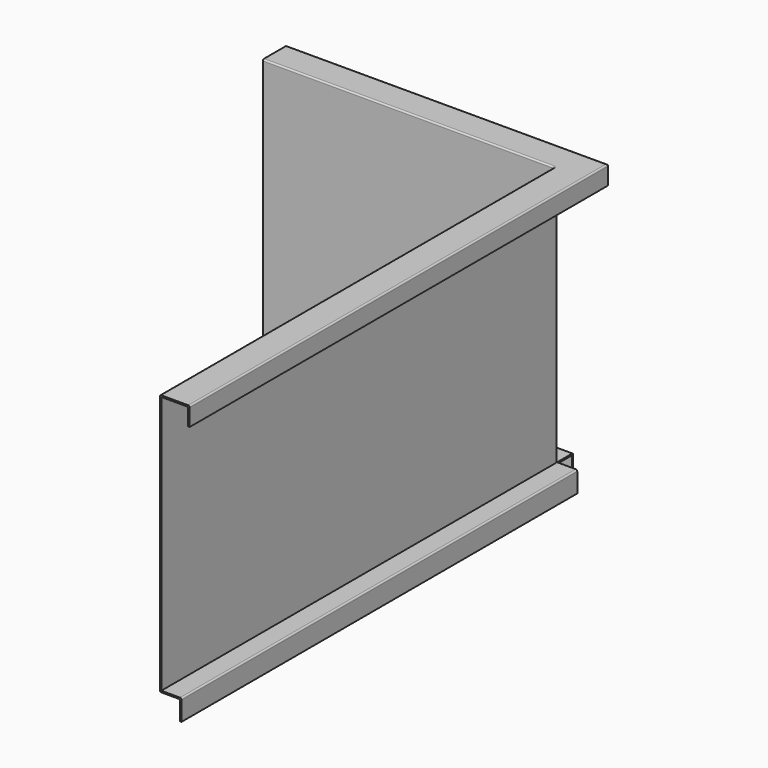
from build123d import *

# Parameters (mm, degrees)
F3_W         = 27
F3_H         = 27
F4_DEPTH     = 30
F5_T1_DEPTH  = 392
F5_T3_DEPTH  = 662
F5_T5_DEPTH  = 350
F5_T10_DEPTH = 703
F5_T15_DEPTH = 433
F5_T17_DEPTH = 672
F5_T19_DEPTH = 402
F5_T21_DEPTH = 440
F5_T23_DEPTH = 710
F5_T25_DEPTH = 346
F5_T27_DEPTH = 660
F5_T29_DEPTH = 390
F5_T32_ANGLE = 90
F5_T33_DEPTH = 663
F5_T35_DEPTH = 393
F5_T38_ANGLE = 90
F5_T40_ANGLE = 90


# Not quite as in the source:
# - a fillet or chamfer that OpenCascade refuses, or shapes differently, is made with other operations: its cross-section is extruded or revolved along the edge and cut away or added


with BuildPart() as f2:
    # F2: sweep along a path in F1
    with BuildLine(Plane.XY) as f2_path:
        Line((0, 0), (0, 660))
        Line((0, 660), (-390, 660))
    # F0 (on Front) → F2 (sweep)
    with BuildSketch(Plane.XZ):
        Polygon((38, -2), (38, -25), (40, -25), (40, 0), (0, 0), (0, -350), (27, -350), (27, -376), (29, -376), (29, -348), (2, -348), (2, -2), align=None)
    sweep(path=f2_path.line, transition=Transition.RIGHT)

    # F3 (on face) → F4 (cut)
    with BuildSketch(Plane.XY.offset(-348)):
        with Locations((15.5, 675.5)):
            Rectangle(F3_W, F3_H)
    extrude(amount=-F4_DEPTH, mode=Mode.SUBTRACT)

    # F5: fillet of radius 2 on 16 edges, made by hand

    # F5_s2 → F5_t1 (join)
    with BuildSketch(Plane.YZ.offset(-390)):
        with BuildLine():
            ThreePointArc((685, -350), (686.4142135624, -350.5857864376), (687, -352))
            Line((687, -352), (687, -350))
            Line((687, -350), (685, -350))
        make_face()
    extrude(amount=F5_T1_DEPTH)

    # F5_s4 → F5_t3 (join)
    with BuildSketch(Plane.XZ.offset(-662)):
        with BuildLine():
            ThreePointArc((25, -350), (26.4142135624, -350.5857864376), (27, -352))
            Line((27, -352), (27, -350))
            Line((27, -350), (25, -350))
        make_face()
    extrude(amount=F5_T3_DEPTH)

    # F5_s6 → F5_t5 (join)
    with BuildSketch(Plane.XY.offset(-350)):
        with BuildLine():
            ThreePointArc((0, 658), (-0.5857864376, 659.4142135624), (-2, 660))
            Line((-2, 660), (0, 660))
            Line((0, 660), (0, 658))
        make_face()
    extrude(amount=F5_T5_DEPTH)


with BuildPart() as f5_tool8:
    # F5_s9 → F5_t10 (new body)
    with BuildSketch(Plane.XZ):
        with BuildLine():
            ThreePointArc((38, -4), (37.4142135624, -2.5857864376), (36, -2))
            Line((36, -2), (38, -2))
            Line((38, -2), (38, -4))
        make_face()
    extrude(amount=-F5_T10_DEPTH)

    split(bisect_by=Plane.XZ.offset(-700), keep=Keep.TOP)


with BuildPart() as f2_1:
    add(f2.part)

    # F5_t7: union F5_tool8
    add(f5_tool8.part)


with BuildPart() as f5_tool13:
    # F5_s14 → F5_t15 (new body)
    with BuildSketch(Plane.YZ.offset(43)):
        with BuildLine():
            ThreePointArc((696, -2), (697.4142135624, -2.5857864376), (698, -4))
            Line((698, -4), (698, -2))
            Line((698, -2), (696, -2))
        make_face()
    extrude(amount=-F5_T15_DEPTH)

    split(bisect_by=Plane.YZ.offset(40), keep=Keep.BOTTOM)


with BuildPart() as f2_2:
    add(f2_1.part)

    # F5_t12: union F5_tool13
    add(f5_tool13.part)

    # F5_s18 → F5_t17 (cut)
    with BuildSketch(Plane.XZ.offset(-667)):
        with BuildLine():
            ThreePointArc((29, -350), (28.4142135624, -348.5857864376), (27, -348))
            Line((27, -348), (29, -348))
            Line((29, -348), (29, -350))
        make_face()
    extrude(amount=F5_T17_DEPTH, mode=Mode.SUBTRACT)

    # F5_s20 → F5_t19 (cut)
    with BuildSketch(Plane.YZ.offset(-395)):
        with BuildLine():
            ThreePointArc((689, -350), (688.4142135624, -348.5857864376), (687, -348))
            Line((687, -348), (689, -348))
            Line((689, -348), (689, -350))
        make_face()
    extrude(amount=F5_T19_DEPTH, mode=Mode.SUBTRACT)

    # F5_s22 → F5_t21 (cut)
    with BuildSketch(Plane.YZ.offset(-395)):
        with BuildLine():
            ThreePointArc((700, -2), (699.4142135624, -0.5857864376), (698, 0))
            Line((698, 0), (700, 0))
            Line((700, 0), (700, -2))
        make_face()
    extrude(amount=F5_T21_DEPTH, mode=Mode.SUBTRACT)

    # F5_s24 → F5_t23 (cut)
    with BuildSketch(Plane.XZ.offset(-705)):
        with BuildLine():
            ThreePointArc((40, -2), (39.4142135624, -0.5857864376), (38, 0))
            Line((38, 0), (40, 0))
            Line((40, 0), (40, -2))
        make_face()
    extrude(amount=F5_T23_DEPTH, mode=Mode.SUBTRACT)

    # F5_s26 → F5_t25 (cut)
    with BuildSketch(Plane.XY.offset(-348)):
        with BuildLine():
            ThreePointArc((2, 660), (1.4142135624, 661.4142135624), (0, 662))
            Line((0, 662), (2, 662))
            Line((2, 662), (2, 660))
        make_face()
    extrude(amount=F5_T25_DEPTH, mode=Mode.SUBTRACT)

    # F5_s28 → F5_t27 (join)
    with BuildSketch(Plane.XZ.offset(-660)):
        with BuildLine():
            ThreePointArc((4, -2), (2.5857864376, -2.5857864376), (2, -4))
            Line((2, -4), (2, -2))
            Line((2, -2), (4, -2))
        make_face()
    extrude(amount=F5_T27_DEPTH)

    # F5_s30 → F5_t29 (join)
    with BuildSketch(Plane.YZ.offset(-390)):
        with BuildLine():
            ThreePointArc((664, -2), (662.5857864376, -2.5857864376), (662, -4))
            Line((662, -4), (662, -2))
            Line((662, -2), (664, -2))
        make_face()
    extrude(amount=F5_T29_DEPTH)

    # F5_s31 → F5_t32 (revolve)
    with BuildSketch(Plane.XZ.offset(-660)):
        with BuildLine():
            ThreePointArc((4, -2), (2.5857864376, -2.5857864376), (2, -4))
            Line((2, -4), (2, -2))
            Line((2, -2), (4, -2))
        make_face()
    revolve(axis=Axis((0, 660, -2), (0, 0, 1)), revolution_arc=F5_T32_ANGLE)

    # F5_s34 → F5_t33 (cut)
    with BuildSketch(Plane.XZ.offset(-658)):
        with BuildLine():
            ThreePointArc((2, -350), (0.5857864376, -349.4142135624), (0, -348))
            Line((0, -348), (0, -350))
            Line((0, -350), (2, -350))
        make_face()
        with BuildLine():
            ThreePointArc((0, -2), (0.5857864376, -0.5857864376), (2, 0))
            Line((2, 0), (0, 0))
            Line((0, 0), (0, -2))
        make_face()
    extrude(amount=F5_T33_DEPTH, mode=Mode.SUBTRACT)

    # F5_s36 → F5_t35 (cut)
    with BuildSketch(Plane.YZ.offset(-395)):
        with BuildLine():
            ThreePointArc((662, -350), (660.5857864376, -349.4142135624), (660, -348))
            Line((660, -348), (660, -350))
            Line((660, -350), (662, -350))
        make_face()
        with BuildLine():
            ThreePointArc((662, 0), (660.5857864376, -0.5857864376), (660, -2))
            Line((660, -2), (660, 0))
            Line((660, 0), (662, 0))
        make_face()
    extrude(amount=F5_T35_DEPTH, mode=Mode.SUBTRACT)

    # F5_s37 → F5_t38 (revolve, cut)
    with BuildSketch(Plane.XZ.offset(-658)):
        with BuildLine():
            ThreePointArc((2, 0), (0.5857864376, -0.5857864376), (0, -2))
            Line((0, -2), (0, 0))
            Line((0, 0), (2, 0))
        make_face()
    revolve(axis=Axis((-2, 658, 0), (0, 0, 1)), revolution_arc=F5_T38_ANGLE, mode=Mode.SUBTRACT)

    # F5_s39 → F5_t40 (revolve, cut)
    with BuildSketch(Plane.XZ.offset(-658)):
        with BuildLine():
            ThreePointArc((2, -350), (0.5857864376, -349.4142135624), (0, -348))
            Line((0, -348), (0, -350))
            Line((0, -350), (2, -350))
        make_face()
    revolve(axis=Axis((-2, 658, -350), (0, 0, 1)), revolution_arc=F5_T40_ANGLE, mode=Mode.SUBTRACT)


solid = f2_2.part
